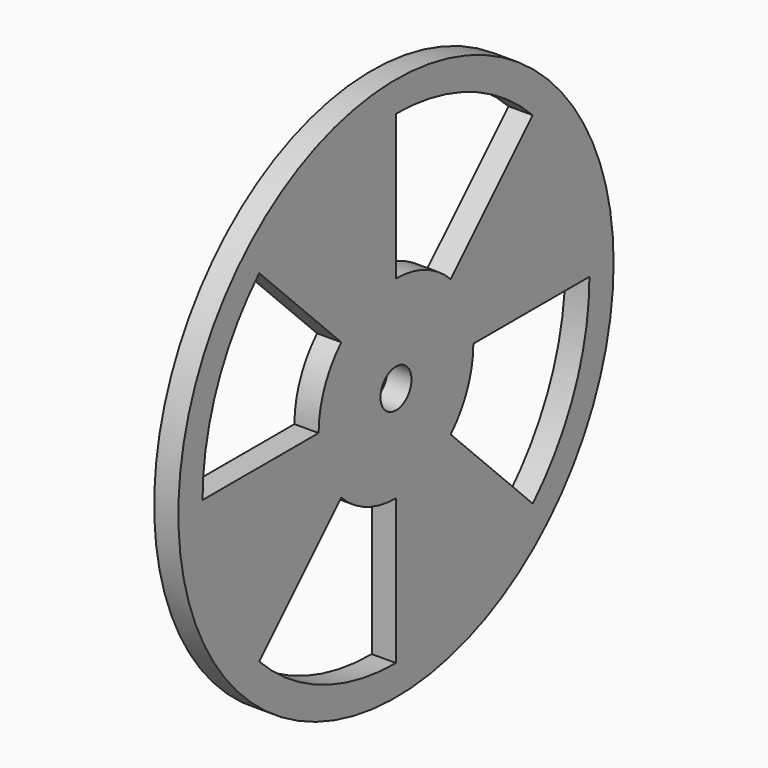
from build123d import *

# Parameters (mm, degrees)
F0_R     = 35.71875
F0_R_2   = 2.54
F1_DEPTH = 3.175


# Not quite as in the source:
# - a length typed as a fraction of an inch, garbled in the dataset ("3 / 203.2 mm" for 3/8 in), is restored


with BuildPart() as f1:
    # F0 (on Right) → F1 (new body)
    with BuildSketch(Plane.YZ):
        Circle(F0_R)
        with BuildLine():
            ThreePointArc((0, -31.75), (-12.1501989776, -29.3331751572), (-22.4506403027, -22.4506403027))
            Line((-22.4506403027, -22.4506403027), (-8.9802561211, -8.9802561211))
            ThreePointArc((-8.9802561211, -8.9802561211), (-4.860079591, -11.7332700629), (0, -12.7))
            Line((0, -12.7), (0, -31.75))
        make_face(mode=Mode.SUBTRACT)
        with BuildLine():
            ThreePointArc((8.9802561211, -8.9802561211), (11.7332700629, -4.860079591), (12.7, 0))
            Line((12.7, 0), (31.75, 0))
            ThreePointArc((31.75, 0), (29.3331751572, -12.1501989776), (22.4506403027, -22.4506403027))
            Line((22.4506403027, -22.4506403027), (8.9802561211, -8.9802561211))
        make_face(mode=Mode.SUBTRACT)
        with BuildLine():
            ThreePointArc((-8.9802561211, 8.9802561211), (-11.7332700629, 4.860079591), (-12.7, 0))
            Line((-12.7, 0), (-31.75, 0))
            ThreePointArc((-31.75, 0), (-29.3331751572, 12.1501989776), (-22.4506403027, 22.4506403027))
            Line((-22.4506403027, 22.4506403027), (-8.9802561211, 8.9802561211))
        make_face(mode=Mode.SUBTRACT)
        Circle(F0_R_2, mode=Mode.SUBTRACT)
        with BuildLine():
            ThreePointArc((8.9802561211, 8.9802561211), (4.860079591, 11.7332700629), (0, 12.7))
            Line((0, 12.7), (0, 31.75))
            ThreePointArc((0, 31.75), (12.1501989776, 29.3331751572), (22.4506403027, 22.4506403027))
            Line((22.4506403027, 22.4506403027), (8.9802561211, 8.9802561211))
        make_face(mode=Mode.SUBTRACT)
    extrude(amount=F1_DEPTH)


solid = f1.part
